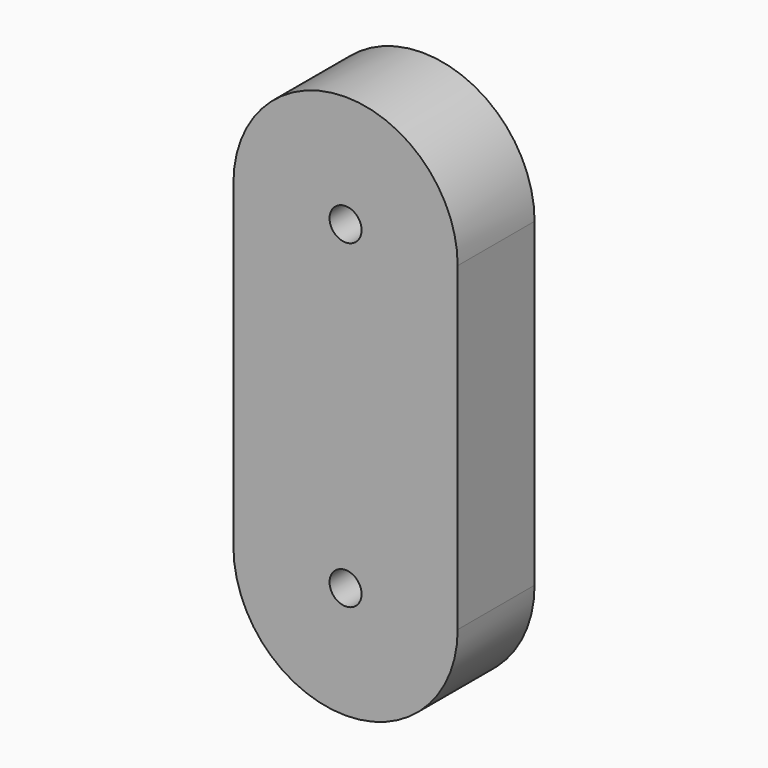
from build123d import *

# Parameters (mm, degrees)
F1_DEPTH = 38.1
F2_D     = 12.7


# Not quite as in the source:
# - a length typed as a fraction of an inch, garbled in the dataset ("3 / 203.2 mm" for 3/8 in), is restored


with BuildPart() as f1:
    # F0 (on Front) → F1 (new body)
    with BuildSketch(Plane.XZ):
        with BuildLine():
            Line((44.45, -63.5), (44.45, 63.5))
            ThreePointArc((44.45, 63.5), (0, 107.95), (-44.45, 63.5))
            Line((-44.45, 63.5), (-44.45, -63.5))
            ThreePointArc((-44.45, -63.5), (0, -107.95), (44.45, -63.5))
        make_face()
    extrude(amount=F1_DEPTH)

    # F2 (through all)
    with Locations(Plane(origin=(0, 0, 0), x_dir=(1, 0, 0), z_dir=(0, 1, 0))):
        with Locations((0, -63.5), (0, 63.5)):
            Hole(F2_D / 2)


solid = f1.part
